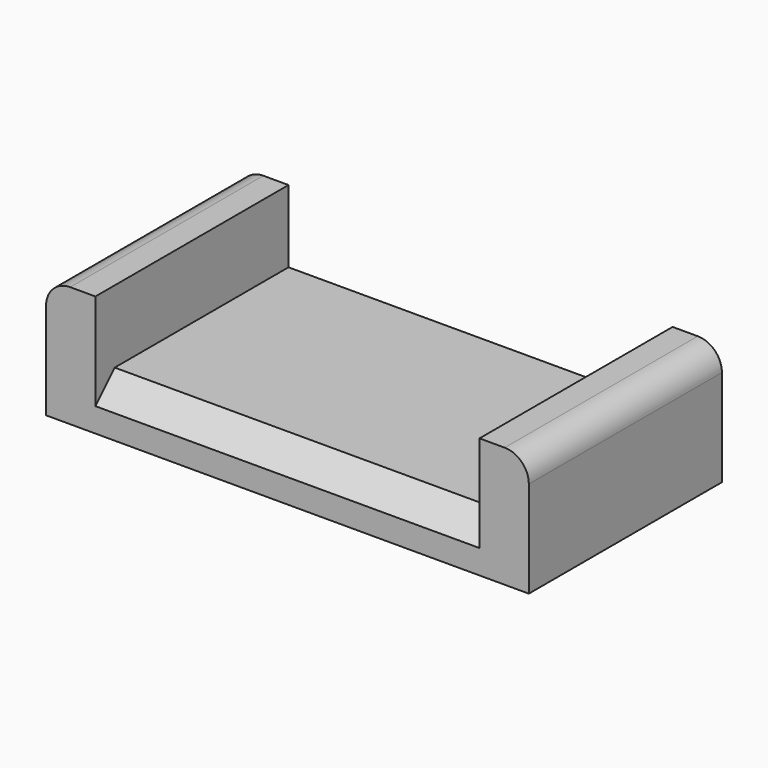
from build123d import *

# Parameters (mm, degrees)
F0_W     = 10.2165445685
F0_H     = 50
F1_DEPTH = 25
F0_W_2   = 79.5669108629
F2_DEPTH = 10
F3_DEPTH = 25
F4_R     = 5
F5_R     = 5
F6_SIZE  = 5


with BuildPart() as f1:
    # F0 (on Top) → F1 (new body)
    with BuildSketch(Plane.XY):
        with Locations((-44.8917277157, 0)):
            Rectangle(F0_W, F0_H)
    extrude(amount=F1_DEPTH)

    # F0 (on Top) → F2 (join)
    with BuildSketch(Plane.XY):
        Rectangle(F0_W_2, F0_H)
    extrude(amount=F2_DEPTH)

    # F0 (on Top) → F3 (join)
    with BuildSketch(Plane.XY):
        with Locations((44.8917277157, 0)):
            Rectangle(F0_W, F0_H)
    extrude(amount=F3_DEPTH)

    # F4
    f4_edges = [f1.edges().sort_by_distance(p)[0] for p in [
        (50, 0, 25),
    ]]
    fillet(f4_edges, radius=F4_R)

    # F5
    f5_edges = [f1.edges().sort_by_distance(p)[0] for p in [
        (-50, 0, 25),
    ]]
    fillet(f5_edges, radius=F5_R)

    # F6
    f6_edges = [f1.edges().sort_by_distance(p)[0] for p in [
        (0, -25, 10),
    ]]
    chamfer(f6_edges, length=F6_SIZE)


solid = f1.part
